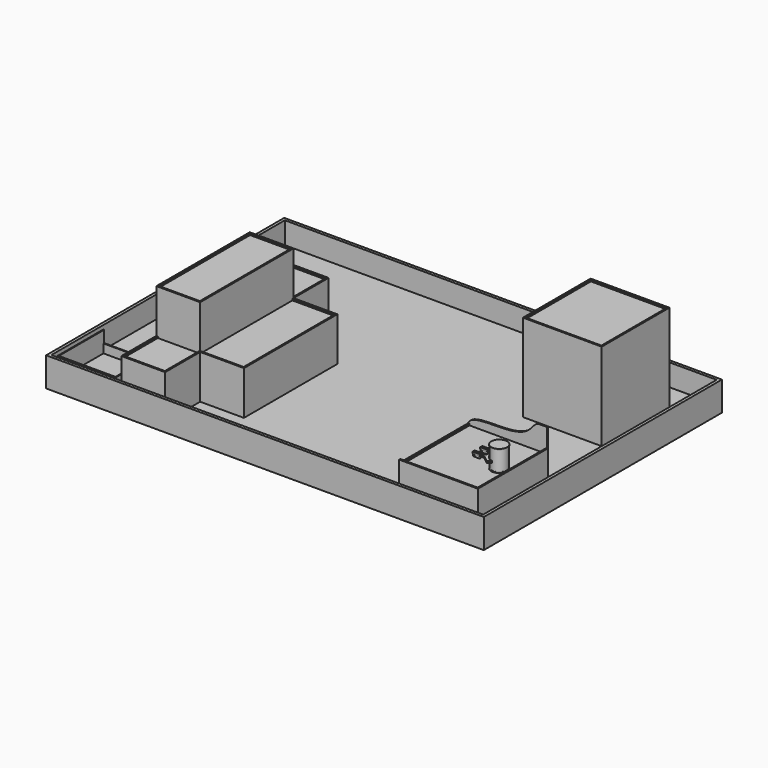
from build123d import *

# Parameters (mm, degrees)
F0_R      = 27.2
F1_DEPTH  = 2.83
F2_R      = 26.4
F3_DEPTH  = 67.36
F4_R      = 27.2
F5_DEPTH  = 2.83
F9_W      = 270
F9_H      = 300
F10_DEPTH = 72
F12_DEPTH = 15
F14_DEPTH = 5
F15_W     = 5
F15_H     = 290
F16_DEPTH = 5
F17_W     = 1500
F17_H     = 1020
F18_DEPTH = 25
F19_W     = 270
F19_H     = 290
F20_DEPTH = 300
F21_W     = 260
F21_H     = 280
F22_DEPTH = 5
F23_W     = 1500
F23_H     = 1020
F23_W_2   = 1480
F23_H_2   = 1000
F24_DEPTH = 75
F26_DEPTH = 150
F27_W     = 150
F27_H     = 400
F28_DEPTH = 150
F29_W     = 140
F29_H     = 390
F30_DEPTH = 5
F31_W     = 140
F31_H     = 145
F31_W_2   = 145
F31_H_2   = 390
F32_DEPTH = 5
F33_R     = 3
F34_DEPTH = 4
F35_R     = 3.99999
F35_2_R   = 3.99999
F36_R     = 3
F37_DEPTH = 8
F38_R     = 3
F39_DEPTH = 8
F40_R     = 3
F40_R_2   = 2.5
F41_DEPTH = 3
F42_R     = 3
F42_R_2   = 2.5
F43_DEPTH = 3
F45_DEPTH = 270.001
F46_W     = 200
F46_H     = 200
F46_W_2   = 194
F46_H_2   = 191
F47_DEPTH = 30
F49_DEPTH = 40
F50_R     = 2.25
F51_DEPTH = 6


# Not quite as in the source:
# - a fillet or chamfer is up to 0.001 mm smaller than in the source, because OpenCascade refuses the exact size
# - a feature names something its author has since deleted; it is built from what else it names


with BuildPart() as f1:
    # F0 (on Top) → F1 (new body)
    with BuildSketch(Plane.XY):
        Circle(F0_R)
    extrude(amount=F1_DEPTH)

    # F2 (on face) → F3 (join)
    with BuildSketch(Plane.XY.offset(2.83)):
        Circle(F2_R)
    extrude(amount=F3_DEPTH)

    # F4 (on face) → F5 (join)
    with BuildSketch(Plane.XY.offset(70.19)):
        Circle(F4_R)
    extrude(amount=F5_DEPTH)


with BuildPart() as f10:
    # F9 (on Top) → F10 (new body)
    with BuildSketch(Plane.XY):
        with Locations((-87.8, 0)):
            Rectangle(F9_W, F9_H)
    extrude(amount=-F10_DEPTH)

    # F11 (on face) → F12 (join)
    with BuildSketch(Plane.XY):
        Polygon((-222.8, -145), (-222.8, -150), (47.2, -150), (47.2, 150), (42.2, 150), (42.2, -145), align=None)
    extrude(amount=F12_DEPTH)

    # F13 (on face) → F14 (join)
    with BuildSketch(Plane(origin=(0, 150, 0), x_dir=(-1, 0, 0), z_dir=(0, 1, 0))):
        with BuildLine():
            Line((-21.3134280931, 81.3575685024), (-47.2, 81.3575685024))
            Line((-47.2, 81.3575685024), (-47.2, -72))
            Line((-47.2, -72), (222.8, -72))
            Line((222.8, -72), (222.8, 0))
            add(Edge.make_bspline(
                [(-21.3134280931, 81.3575685024), (-6.3059147253, 81.3822787863), (12.9585432644, 38.1268753575), (103.6097013063, 23.6068887567), (223.0224295336, 30.7718731823), (222.8, 0)],
                knots=[0, 0, 0, 0, 0.2487100673, 0.6151112321, 1, 1, 1, 1], degree=3))
        make_face()
    extrude(amount=-F14_DEPTH)

    # F15 (on face) → F16 (join)
    with BuildSketch(Plane.XY):
        with Locations((-220.3, 0)):
            Rectangle(F15_W, F15_H)
    extrude(amount=F16_DEPTH)

    # F17 (on face) → F18 (join)
    with BuildSketch(Plane(origin=(0, 0, -72), x_dir=(1, 0, 0), z_dir=(0, 0, -1))):
        with Locations((-602.8, -260)):
            Rectangle(F17_W, F17_H)
    extrude(amount=F18_DEPTH)

    # F19 (on face) → F20 (join)
    with BuildSketch(Plane.XY.offset(-72)):
        with Locations((-87.8, 525)):
            Rectangle(F19_W, F19_H)
    extrude(amount=F20_DEPTH)

    # F21 (on face) → F22 (cut)
    with BuildSketch(Plane.XY.offset(228)):
        with Locations((-87.8, 525)):
            Rectangle(F21_W, F21_H)
    extrude(amount=-F22_DEPTH, mode=Mode.SUBTRACT)

    # F23 (on face) → F24 (join)
    with BuildSketch(Plane.XY.offset(-72)):
        with Locations((-602.8, 260)):
            Rectangle(F23_W, F23_H)
        with Locations((-602.8, 260)):
            Rectangle(F23_W_2, F23_H_2, mode=Mode.SUBTRACT)
    extrude(amount=F24_DEPTH)

    # F25 (on face) → F26 (join)
    with BuildSketch(Plane.XY.offset(-72)):
        Polygon((-952.8, 460), (-1102.8, 460), (-1102.8, -240), (-952.8, -240), (-952.8, -90), (-802.8, -90), (-802.8, 310), (-952.8, 310), align=None)
    extrude(amount=F26_DEPTH)

    # F27 (on face) → F28 (join)
    with BuildSketch(Plane.XY.offset(78)):
        with Locations((-1027.8, 110)):
            Rectangle(F27_W, F27_H)
    extrude(amount=F28_DEPTH)

    # F29 (on face) → F30 (cut)
    with BuildSketch(Plane.XY.offset(228)):
        with Locations((-1027.8, 110)):
            Rectangle(F29_W, F29_H)
    extrude(amount=-F30_DEPTH, mode=Mode.SUBTRACT)

    # F31 (on face) → F32 (cut)
    with BuildSketch(Plane.XY.offset(78)):
        with Locations((-1027.8, 382.5)):
            Rectangle(F31_W, F31_H)
        with Locations((-880.3, 110)):
            Rectangle(F31_W_2, F31_H_2)
        with Locations((-1027.8, -162.5)):
            Rectangle(F31_W, F31_H)
    extrude(amount=-F32_DEPTH, mode=Mode.SUBTRACT)

    # F46 (on face) → F47 (join)
    with BuildSketch(Plane.XY.offset(-72)):
        with Locations((-1232.8, -130)):
            Rectangle(F46_W, F46_H)
        with Locations((-1232.8, -128.5)):
            Rectangle(F46_W_2, F46_H_2, mode=Mode.SUBTRACT)
    extrude(amount=F47_DEPTH)

    # F48 (on face) → F49 (join)
    with BuildSketch(Plane.XY.offset(-42)):
        Polygon((-1329.8, -30), (-1332.8, -30), (-1332.8, -230), (-1329.8, -230), (-1135.8, -230), (-1132.8, -230), (-1132.8, -30), (-1135.8, -30), (-1135.8, -224), (-1329.8, -224), align=None)
    extrude(amount=F49_DEPTH)


with BuildPart() as f34:
    # F33 (on offset) → F34 (new body, symmetric)
    with BuildSketch(Plane.XY.offset(25)):
        with BuildLine():
            Line((-55, -12), (-74.5, -12))
            Line((-74.5, -12), (-74.5, -13))
            Line((-74.5, -13), (-65.6457513111, -13))
            ThreePointArc((-65.6457513111, -13), (-67, -16), (-65.6457513111, -19))
            Line((-65.6457513111, -19), (-74.5, -19))
            Line((-74.5, -19), (-74.5, -20))
            Line((-74.5, -20), (-55, -20))
            ThreePointArc((-55, -20), (-51, -16), (-55, -12))
        make_face()
        with Locations((-63, -16)):
            Circle(F33_R, mode=Mode.SUBTRACT)
        with Locations((-55, -16)):
            Circle(F33_R, mode=Mode.SUBTRACT)
    extrude(amount=F34_DEPTH, both=True)

    # F35 (radius 4 in the source; OpenCascade refuses exactly that, so slightly less here)
    f35_edges = [f34.edges().sort_by_distance(p)[0] for p in [
        (-74.5, -19.5, 29),
        (-74.5, -12.5, 29),
        (-74.5, -19.5, 21),
        (-74.5, -12.5, 21),
    ]]
    fillet(f35_edges, radius=F35_R)

    # F36 (on face) → F37 (join, through all)
    with BuildSketch(Plane.XZ.offset(20)):
        with Locations((-70.5, 25)):
            Circle(F36_R)
    extrude(amount=-F37_DEPTH)

    # F42 (on offset) → F43 (join, symmetric)
    with BuildSketch(Plane.XY.offset(25)):
        with Locations((-63, -16)):
            Circle(F42_R)
        with Locations((-63, -16)):
            Circle(F42_R_2, mode=Mode.SUBTRACT)
        with Locations((-55, -16)):
            Circle(F42_R)
        with Locations((-55, -16)):
            Circle(F42_R_2, mode=Mode.SUBTRACT)
    extrude(amount=F43_DEPTH, both=True)


with BuildPart() as f34b:
    # F33 (on offset) → F34, piece 2 (new body, symmetric)
    with BuildSketch(Plane.XY.offset(25)):
        with BuildLine():
            Line((-74.5, 13), (-74.5, 12))
            Line((-74.5, 12), (-55, 12))
            ThreePointArc((-55, 12), (-51, 16), (-55, 20))
            Line((-55, 20), (-74.5, 20))
            Line((-74.5, 20), (-74.5, 19))
            Line((-74.5, 19), (-65.6457513111, 19))
            ThreePointArc((-65.6457513111, 19), (-67, 16), (-65.6457513111, 13))
            Line((-65.6457513111, 13), (-74.5, 13))
        make_face()
        with Locations((-63, 16)):
            Circle(F33_R, mode=Mode.SUBTRACT)
        with Locations((-55, 16)):
            Circle(F33_R, mode=Mode.SUBTRACT)
    extrude(amount=F34_DEPTH, both=True)

    # F35#2 (radius 4 in the source; OpenCascade refuses exactly that, so slightly less here)
    f35_2_edges = [f34b.edges().sort_by_distance(p)[0] for p in [
        (-74.5, 12.5, 29),
        (-74.5, 19.5, 29),
        (-74.5, 19.5, 21),
        (-74.5, 12.5, 21),
    ]]
    fillet(f35_2_edges, radius=F35_2_R)

    # F38 (on face) → F39 (join, through all)
    with BuildSketch(Plane(origin=(0, 20, 0), x_dir=(-1, 0, 0), z_dir=(0, 1, 0))):
        with Locations((70.5, 25)):
            Circle(F38_R)
    extrude(amount=-F39_DEPTH)

    # F40 (on offset) → F41 (join, symmetric)
    with BuildSketch(Plane.XY.offset(25)):
        with Locations((-55, 16)):
            Circle(F40_R)
        with Locations((-55, 16)):
            Circle(F40_R_2, mode=Mode.SUBTRACT)
        with Locations((-63, 16)):
            Circle(F40_R)
        with Locations((-63, 16)):
            Circle(F40_R_2, mode=Mode.SUBTRACT)
    extrude(amount=F41_DEPTH, both=True)


with BuildPart() as f45_tool:
    # F44 (on face) → F45 (new body, through all)
    with BuildSketch(Plane(origin=(0, 20, 0), x_dir=(-1, 0, 0), z_dir=(0, 1, 0))):
        with BuildLine():
            Line((71.5, 26), (71.5, 27.2912878475))
            ThreePointArc((71.5, 27.2912878475), (70.5, 27.5), (69.5, 27.2912878475))
            Line((69.5, 27.2912878475), (69.5, 26))
            Line((69.5, 26), (68.2087121525, 26))
            ThreePointArc((68.2087121525, 26), (68, 25), (68.2087121525, 24))
            Line((68.2087121525, 24), (69.5, 24))
            Line((69.5, 24), (69.5, 22.7087121525))
            ThreePointArc((69.5, 22.7087121525), (70.5, 22.5), (71.5, 22.7087121525))
            Line((71.5, 22.7087121525), (71.5, 24))
            Line((71.5, 24), (72.7912878475, 24))
            ThreePointArc((72.7912878475, 24), (73, 25), (72.7912878475, 26))
            Line((72.7912878475, 26), (71.5, 26))
        make_face()
    extrude(amount=-F45_DEPTH)


with BuildPart() as f34_1:
    add(f34.part)

    # F45: cut by f45_tool
    add(f45_tool.part, mode=Mode.SUBTRACT)


with BuildPart() as f34b_1:
    add(f34b.part)

    # F45: cut by f45_tool
    add(f45_tool.part, mode=Mode.SUBTRACT)


with BuildPart() as f51:
    # F50 (on face) → F51 (new body)
    with BuildSketch(Plane.XY.offset(29)):
        with BuildLine():
            ThreePointArc((-0.8694231288, -29.9651682592), (-27.1097646961, -0.16589585), (-0.8829690239, 29.6452992025))
            Line((-0.8829690239, 29.6452992025), (-10.4092834421, 39.9044089887))
            Line((-10.4092834421, 39.9044089887), (-34.7385093788, 20.6927259462))
            Line((-34.7385093788, 20.6927259462), (-74.7385093788, 20.6927259462))
            Line((-74.7385093788, 20.6927259462), (-74.7385093788, 11.6927259462))
            Line((-74.7385093788, 11.6927259462), (-34.7385093788, 11.6927259462))
            Line((-34.7385093788, 11.6927259462), (-34.7385093788, -12))
            Line((-34.7385093788, -12), (-74.7385093788, -12))
            Line((-74.7385093788, -12), (-74.7385093788, -21))
            Line((-74.7385093788, -21), (-34.7385093788, -21))
            Line((-34.7385093788, -21), (-10.4092834421, -40.2116830424))
            Line((-10.4092834421, -40.2116830424), (-0.8694231288, -29.9651682592))
        make_face()
        with Locations((-63, -16)):
            Circle(F50_R, mode=Mode.SUBTRACT)
        with Locations((-55, -16)):
            Circle(F50_R, mode=Mode.SUBTRACT)
        with Locations((-62.9937574267, 16.0129591823)):
            Circle(F50_R, mode=Mode.SUBTRACT)
        with Locations((-55.0742894411, 16.050670296)):
            Circle(F50_R, mode=Mode.SUBTRACT)
    extrude(amount=F51_DEPTH)


solid = Compound([f1.part, f10.part, f34_1.part, f34b_1.part, f51.part])
